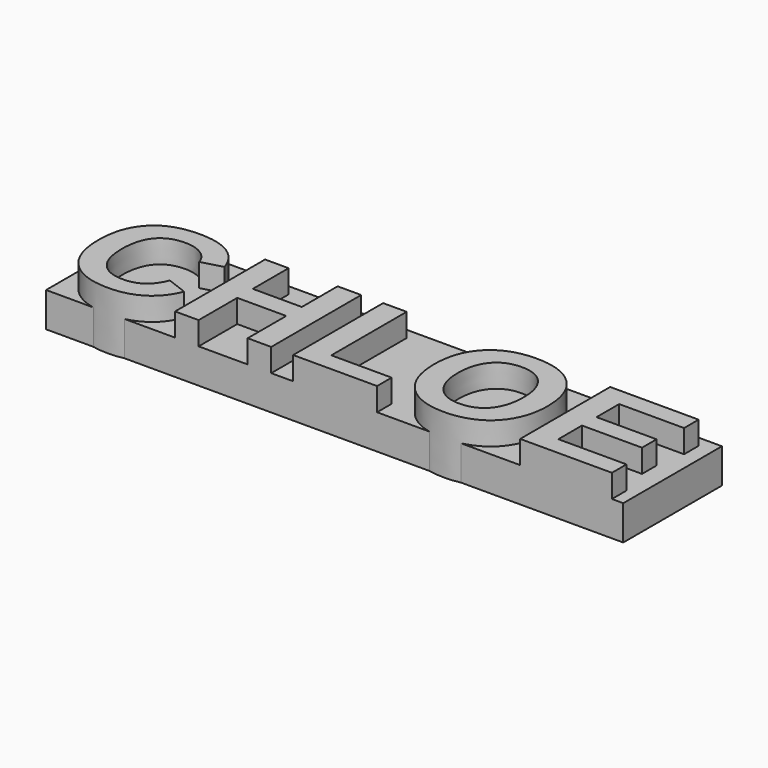
from build123d import *

# Parameters (mm, degrees)
F1_W         = 63.5
F1_H         = 13.5702025145
F2_DEPTH     = 3.81
F0_TEXT_SIZE = 17.9870762149
F3_DEPTH     = 6.35


# Not quite as in the source:
# - Text() gives the source's letters only with a copy of the font that has no kerning and outlines rounded to 1/6400 em; it was checked with that copy


with BuildPart() as f2:
    # F1 (on Top) → F2 (new body)
    with BuildSketch(Plane.XY):
        with Locations((31.75, 6.7851012573)):
            Rectangle(F1_W, F1_H)
    extrude(amount=F2_DEPTH)

    # F0 (on Top) → F3 (join)
    with BuildSketch(Plane.XY):
        with Locations((0, 0)):
            Text('CHLOE', F0_TEXT_SIZE, font='Arimo', font_style=FontStyle.BOLD, text_align=(TextAlign.LEFT, TextAlign.BOTTOM))
    extrude(amount=F3_DEPTH)


solid = f2.part
